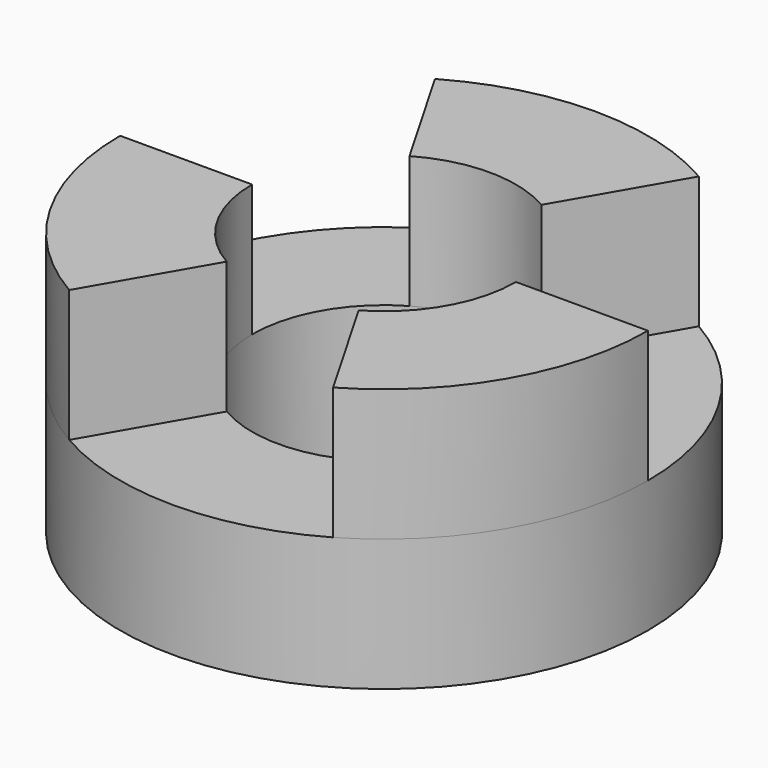
from build123d import *
from build123d import SkipClean  # not in build123d's __all__

# Parameters (mm, degrees)
F0_R     = 10
F0_R_2   = 5
F1_DEPTH = 5
F3_DEPTH = 5


with BuildPart() as f1:
    # F0 (on Top) → F1 (new body)
    with BuildSketch(Plane.XY):
        Circle(F0_R)
        Circle(F0_R_2, mode=Mode.SUBTRACT)
    extrude(amount=F1_DEPTH)

    # F2 (on face) → F3 (join)
    with BuildSketch(Plane.XY.offset(5)):
        with BuildLine():
            ThreePointArc((-2.5, -4.3301270189), (-4.3301270189, -2.5), (-5, 0))
            Line((-5, 0), (-10, 0))
            ThreePointArc((-10, 0), (-8.6602540378, -5), (-5, -8.6602540378))
            Line((-5, -8.6602540378), (-2.5, -4.3301270189))
        make_face()
        with BuildLine():
            ThreePointArc((5, 0), (4.3301270189, -2.5), (2.5, -4.3301270189))
            Line((2.5, -4.3301270189), (5, -8.6602540378))
            ThreePointArc((5, -8.6602540378), (8.6602540378, -5), (10, 0))
            Line((10, 0), (5, 0))
        make_face()
        with BuildLine():
            ThreePointArc((-2.5, 4.3301270189), (0, 5), (2.5, 4.3301270189))
            Line((2.5, 4.3301270189), (5, 8.6602540378))
            ThreePointArc((5, 8.6602540378), (0, 10), (-5, 8.6602540378))
            Line((-5, 8.6602540378), (-2.5, 4.3301270189))
        make_face()
    with SkipClean():  # cleaning this boolean's faces spoils the solid; the shape is the same uncleaned
        extrude(amount=F3_DEPTH)


solid = f1.part
